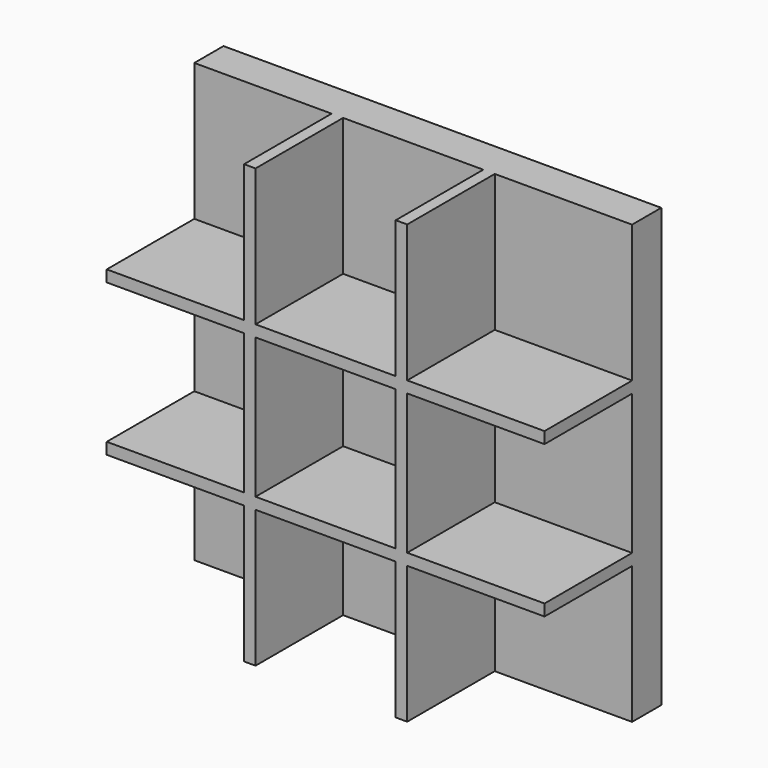
from build123d import *

# Parameters (mm, degrees)
F0_W     = 76.2
F0_H     = 76.2
F3_DEPTH = 6.35
F6_E7_W  = 76.2
F6_E7_H  = 25.4
F7_DEPTH = 2.00000108
F6_E9_W  = 76.2
F6_E9_H  = 25.4
F8_DEPTH = 2.00000108
F5_E11_W = 76.2
F5_E11_H = 25.4
F5_E5_W  = 76.2
F5_E5_H  = 25.4
F9_DEPTH = 2.00000108


# Not quite as in the source:
# - the program builds the solid bodies; features that only make, move or delete a surface that nothing else refers to are left out


with BuildPart() as f3:
    # F0 (on Front) → F3 (new body)
    with BuildSketch(Plane.XZ):
        with Locations((-0.0921785831, 11.5903750752)):
            Rectangle(F0_W, F0_H)
    extrude(amount=F3_DEPTH)

    # F6_E7 (on explicit) → F7 (join)
    with BuildSketch(Plane(origin=(-38.1921785831, 0, 25.7983756152), x_dir=(1, 0, 0), z_dir=(0, 0, -1))):
        with Locations((38.1, 12.7)):
            Rectangle(F6_E7_W, F6_E7_H)
    extrude(amount=F7_DEPTH)

    # F6_E9 (on explicit) → F8 (join)
    with BuildSketch(Plane(origin=(-38.1921785831, 0, -0.6176243848), x_dir=(1, 0, 0), z_dir=(0, 0, -1))):
        with Locations((38.1, 12.7)):
            Rectangle(F6_E9_W, F6_E9_H)
    extrude(amount=F8_DEPTH)

    # F5_E11 (on explicit) + F5_E5 (on explicit) → F9 (join)
    with BuildSketch(Plane(origin=(-12.2921770431, 0, 49.6903750752), x_dir=(0, 0, -1), z_dir=(-1, 0, 0))):
        with Locations((38.1, 12.7)):
            Rectangle(F5_E11_W, F5_E11_H)
    with BuildSketch(Plane(origin=(14.1078209569, 0, 49.6903750752), x_dir=(0, 0, -1), z_dir=(-1, 0, 0))):
        with Locations((38.1, 12.7)):
            Rectangle(F5_E5_W, F5_E5_H)
    extrude(amount=F9_DEPTH)


solid = f3.part
